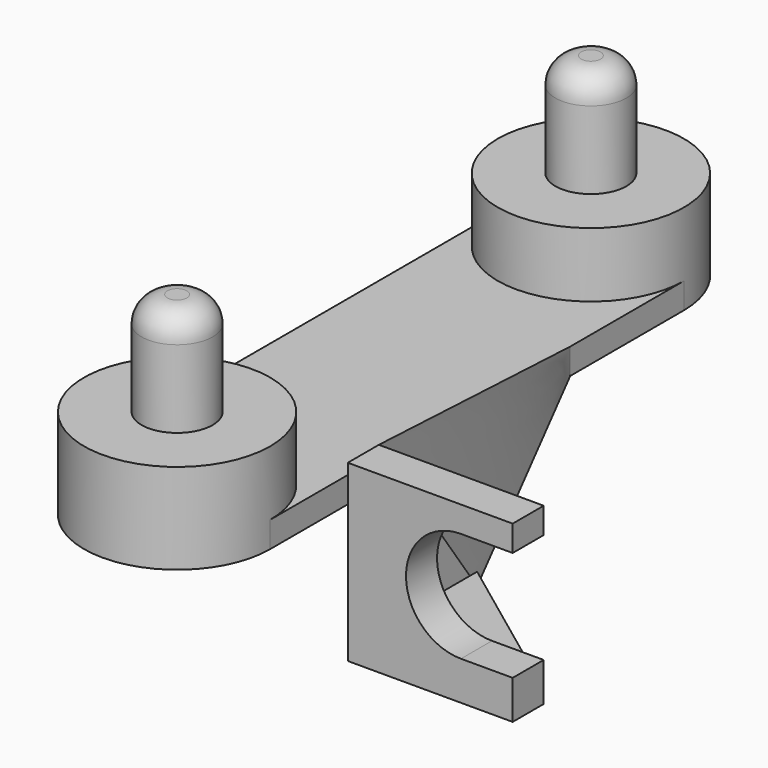
from build123d import *

# Parameters (mm, degrees)
F1_DEPTH  = 2
F2_R      = 2.75
F3_DEPTH  = 13
F6_DEPTH  = 3
F8_W      = 20
F8_H      = 2
F11_DEPTH = 1
F13_DEPTH = 5
F14_R     = 2


with BuildPart() as f1:
    # F0 (on Top) → F1 (new body)
    with BuildSketch(Plane.XY):
        with BuildLine():
            ThreePointArc((7.2, 20), (0, 27.2), (-7.2, 20))
            Line((-7.2, 20), (-7.2, -20))
            ThreePointArc((-7.2, -20), (0, -27.2), (7.2, -20))
            Line((7.2, -20), (7.2, 20))
        make_face()
    extrude(amount=F1_DEPTH)

    # F2 (on face) → F3 (join)
    with BuildSketch(Plane.XY.offset(2)):
        with Locations((0, 20)):
            Circle(F2_R)
        with Locations((0, -20)):
            Circle(F2_R)
    extrude(amount=F3_DEPTH)



with BuildPart() as f6:
    # F5 (on offset) → F6 (new body)
    with BuildSketch(Plane.XZ.offset(28.5)):
        with BuildLine():
            Line((20, 0), (32.75, 0))
            Line((32.75, 0), (32.75, 3))
            Line((32.75, 3), (28.75, 3))
            ThreePointArc((28.75, 3), (24.5, 7.25), (28.75, 11.5))
            Line((28.75, 11.5), (32.75, 11.5))
            Line((32.75, 11.5), (32.75, 13.5))
            Line((32.75, 13.5), (20, 13.5))
            Line((20, 13.5), (20, 0))
        make_face()
    extrude(amount=-F6_DEPTH)


with BuildPart() as f1_1:
    add(f1.part)

    add(f6.part)  # F9 merges F6
    # F7 (on face) → F9 section 0
    with BuildSketch(Plane(origin=(20, 0, 0), x_dir=(0, -1, 0), z_dir=(-1, 0, 0))):
        Polygon((16, 0), (28.5, 0), (28.5, 13.5), (25.5, 13.5), align=None)
    # F8 (on face) → F9 section 1
    with BuildSketch(Plane.YZ.offset(7.2)):
        with Locations((-1, 1)):
            Rectangle(F8_W, F8_H)
    loft()

    # F10 (on face) → F11 (join)
    with BuildSketch(Plane(origin=(0, 0, 0), x_dir=(1, 0, 0), z_dir=(0, 0, -1))):
        Polygon((20, 16), (32.75, 25.5), (20, 25.5), align=None)
    extrude(amount=-F11_DEPTH)

    # F12 (on face) → F13 (join)
    with BuildSketch(Plane.XY.offset(2)):
        with BuildLine():
            ThreePointArc((7.2, 20), (0, 27.2), (-7.2, 20))
            ThreePointArc((-7.2, 20), (0, 12.8), (7.2, 20))
        make_face()
        with BuildLine():
            ThreePointArc((-7.2, -20), (0, -27.2), (7.2, -20))
            ThreePointArc((7.2, -20), (0, -12.8), (-7.2, -20))
        make_face()
    extrude(amount=F13_DEPTH)

    # F14
    f14_edges = [f1_1.edges().sort_by_distance(p)[0] for p in [
        (-2.75, 20, 15),
        (-2.75, -20, 15),
    ]]
    fillet(f14_edges, radius=F14_R)


solid = f1_1.part
